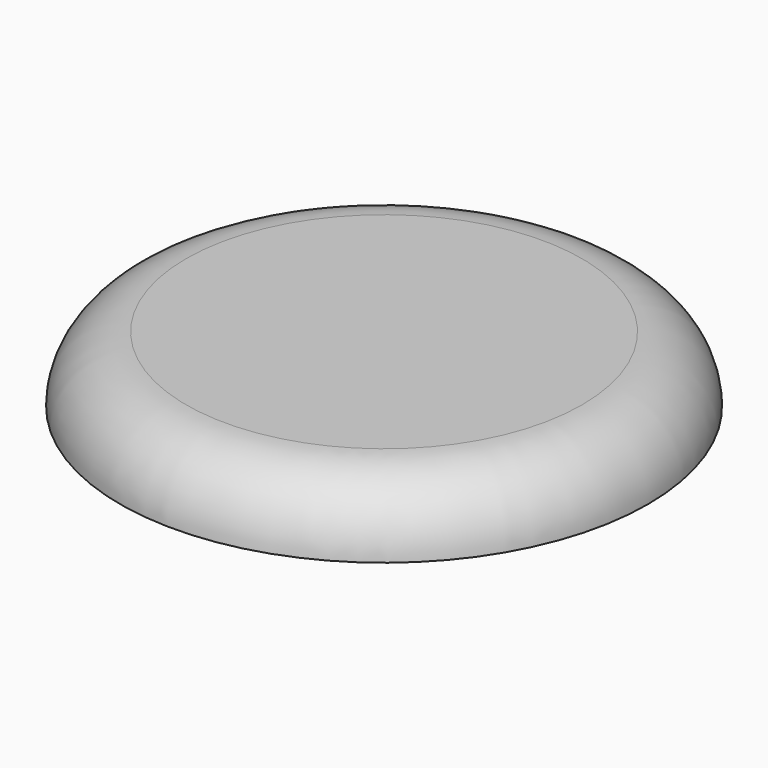
from build123d import *

# Parameters (mm, degrees)
F0_R     = 25.4
F1_DEPTH = 3.175
F2_R     = 6.34999


# Not quite as in the source:
# - a fillet or chamfer is up to 0.001 mm smaller than in the source, because OpenCascade refuses the exact size


with BuildPart() as f1:
    # F0 (on Top) → F1 (new body, symmetric)
    with BuildSketch(Plane.XY):
        Circle(F0_R)
    extrude(amount=F1_DEPTH, both=True)

    # F2 (radius 6.35 in the source; OpenCascade refuses exactly that, so slightly less here)
    f2_edges = [f1.edges().sort_by_distance(p)[0] for p in [
        (-25.4, 0, 3.175),
    ]]
    fillet(f2_edges, radius=F2_R)


solid = f1.part
